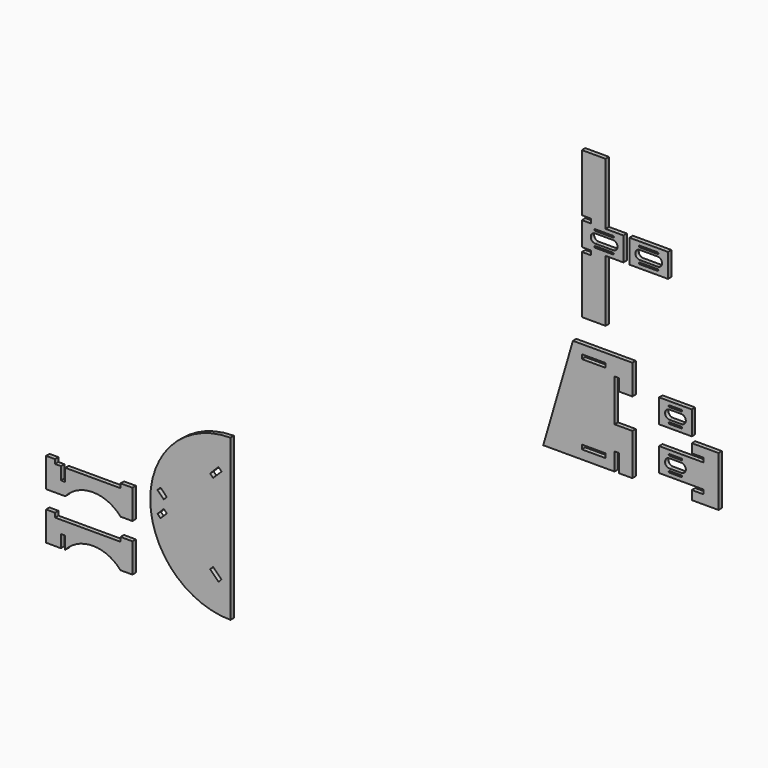
from build123d import *

# Parameters (mm, degrees)
F0_W     = 38.1
F0_H     = 18.288
F0_W_2   = 50.8
F0_W_3   = 18.288
F0_H_2   = 53.594
F1_DEPTH = 18.288
F0_W_4   = 101.6
F0_W_5   = 57.912
F0_H_3   = 76.2
F0_W_6   = 63.5
F0_W_7   = 139.7
F0_H_4   = 101.6
F0_W_8   = 165.1


# Not quite as in the source:
# - a feature names something its author has since deleted; it is built from what else it names


with BuildPart() as f1:
    # F0 (on Front) → F1 (new body)
    with BuildSketch(Plane.XZ):
        with Locations((-2420.2061958742, -155.956)):
            Rectangle(F0_W, F0_H)
        Polygon((-2401.1561958742, -165.1), (-2439.2561958742, -165.1), (-2439.2561958742, -272.288), (-2375.7561958742, -272.288), (-2375.7561958742, -218.694), (-2375.7561958742, -165.1), align=None)
        with BuildLine():
            Line((-2120.9, -165.1), (-2357.4681958742, -165.1))
            Line((-2357.4681958742, -165.1), (-2357.4681958742, -218.694))
            Line((-2357.4681958742, -218.694), (-2357.4681958742, -272.288))
            ThreePointArc((-2357.4681958742, -272.288), (-2239.1840979371, -218.694), (-2120.9, -272.288))
            Line((-2120.9, -272.288), (-2070.1, -272.288))
            Line((-2070.1, -272.288), (-2070.1, -165.1))
            Line((-2070.1, -165.1), (-2120.9, -165.1))
        make_face()
        with Locations((-2095.5, -155.956)):
            Rectangle(F0_W_2, F0_H)
        with Locations((-2366.6121958742, -245.491)):
            Rectangle(F0_W_3, F0_H_2)
    extrude(amount=F1_DEPTH)


with BuildPart() as f1b:
    # F0 (on Front) → F1, piece 2 (new body)
    with BuildSketch(Plane.XZ):
        with BuildLine():
            Line((-1651, -508), (-1651, 177.8))
            ThreePointArc((-1651, 177.8), (-1993.9, -165.1), (-1651, -508))
        make_face()
        Polygon((-1923.1920810565, -195.9920810565), (-1950.1328494197, -222.9328494197), (-1963.064418234, -210.0012806053), (-1936.1236498708, -183.0605122421), align=None, mode=Mode.SUBTRACT)
        Polygon((-1950.1328494197, -107.2671505803), (-1923.1920810565, -134.2079189435), (-1936.1236498708, -147.1394877579), (-1963.064418234, -120.1987193947), align=None, mode=Mode.SUBTRACT)
        Polygon((-1725.0210244843, -332.3789755157), (-1689.1, -368.3), (-1702.0315688143, -381.2315688143), (-1737.9525932986, -345.3105443301), align=None, mode=Mode.SUBTRACT)
        Polygon((-1702.0315688143, 51.0315688143), (-1689.1, 38.1), (-1725.0210244843, 2.1789755157), (-1737.9525932986, 15.1105443301), align=None, mode=Mode.SUBTRACT)
    extrude(amount=F1_DEPTH)


with BuildPart() as f1c:
    # F0 (on Front) → F1, piece 3 (new body)
    with BuildSketch(Plane.XZ):
        with Locations((-2420.2061958742, -357.632)):
            Rectangle(F0_W, F0_H)
        with BuildLine():
            Line((-2120.9, -366.776), (-2357.4681958742, -366.776))
            Line((-2357.4681958742, -366.776), (-2357.4681958742, -420.37))
            Line((-2357.4681958742, -420.37), (-2357.4681958742, -473.964))
            ThreePointArc((-2357.4681958742, -473.964), (-2239.1840979371, -420.37), (-2120.9, -473.964))
            Line((-2120.9, -473.964), (-2070.1, -473.964))
            Line((-2070.1, -473.964), (-2070.1, -366.776))
            Line((-2070.1, -366.776), (-2120.9, -366.776))
        make_face()
        with Locations((-2095.5, -357.632)):
            Rectangle(F0_W_2, F0_H)
        Polygon((-2401.1561958742, -366.776), (-2439.2561958742, -366.776), (-2439.2561958742, -473.964), (-2375.7561958742, -473.964), (-2375.7561958742, -420.37), (-2375.7561958742, -366.776), align=None)
        with Locations((-2366.6121958742, -393.573)):
            Rectangle(F0_W_3, F0_H_2)
    extrude(amount=F1_DEPTH)


with BuildPart() as f1d:
    # F0 (on Front) → F1, piece 4 (new body)
    with BuildSketch(Plane.XZ):
        Polygon((-98.044, 1503.6038), (-47.244, 1503.6038), (-47.244, 1748.8408), (-148.844, 1748.8408), (-148.844, 1503.6038), (-110.744, 1503.6038), align=None)
        Polygon((-98.044, 1485.3158), (-47.244, 1485.3158), (-47.244, 1503.6038), (-98.044, 1503.6038), (-110.744, 1503.6038), (-110.744, 1485.3158), align=None)
        Polygon((-98.044, 1383.7158), (-47.244, 1383.7158), (28.956, 1383.7158), (28.956, 1485.3158), (-47.244, 1485.3158), (-98.044, 1485.3158), (-110.744, 1485.3158), (-148.844, 1485.3158), (-148.844, 1383.7158), (-110.744, 1383.7158), align=None)
        with BuildLine():
            ThreePointArc((-91.694, 1399.4638), (-94.996, 1402.7658), (-91.694, 1406.0678))
            Line((-91.694, 1406.0678), (-15.494, 1406.0678))
            ThreePointArc((-15.494, 1406.0678), (-12.192, 1402.7658), (-15.494, 1399.4638))
            Line((-15.494, 1399.4638), (-91.694, 1399.4638))
        make_face(mode=Mode.SUBTRACT)
        with BuildLine():
            Line((-91.694, 1453.5658), (-15.494, 1453.5658))
            ThreePointArc((-15.494, 1453.5658), (3.556, 1434.5158), (-15.494, 1415.4658))
            Line((-15.494, 1415.4658), (-91.694, 1415.4658))
            ThreePointArc((-91.694, 1415.4658), (-110.744, 1434.5158), (-91.694, 1453.5658))
        make_face(mode=Mode.SUBTRACT)
        with BuildLine():
            Line((-15.494, 1462.9638), (-91.694, 1462.9638))
            ThreePointArc((-91.694, 1462.9638), (-94.996, 1466.2658), (-91.694, 1469.5678))
            Line((-91.694, 1469.5678), (-15.494, 1469.5678))
            ThreePointArc((-15.494, 1469.5678), (-12.192, 1466.2658), (-15.494, 1462.9638))
        make_face(mode=Mode.SUBTRACT)
        Polygon((-98.044, 1365.4278), (-47.244, 1365.4278), (-47.244, 1383.7158), (-98.044, 1383.7158), (-110.744, 1383.7158), (-110.744, 1365.4278), align=None)
        Polygon((-148.844, 1365.4278), (-148.844, 1120.1908), (-47.244, 1120.1908), (-47.244, 1365.4278), (-98.044, 1365.4278), (-110.744, 1365.4278), align=None)
    extrude(amount=F1_DEPTH)


with BuildPart() as f1e:
    # F0 (on Front) → F1, piece 5 (new body)
    with BuildSketch(Plane.XZ):
        Polygon((-9.144, 942.3908), (9.144, 942.3908), (9.144, 929.6908), (9.144, 891.5908), (67.056, 891.5908), (67.056, 929.6908), (67.056, 1018.5908), (-9.144, 1018.5908), (-186.944, 1018.5908), (-313.944, 584.2), (-9.144, 584.2), (-9.144, 660.4), (-9.144, 762), (-9.144, 929.6908), align=None)
        with Locations((-98.044, 631.444)):
            Rectangle(F0_W_4, F0_H, mode=Mode.SUBTRACT)
        with Locations((-98.044, 971.3468)):
            Rectangle(F0_W_4, F0_H, mode=Mode.SUBTRACT)
        Polygon((67.056, 762), (-9.144, 762), (-9.144, 660.4), (9.144, 660.4), (67.056, 660.4), align=None)
        with Locations((38.1, 622.3)):
            Rectangle(F0_W_5, F0_H_3)
    extrude(amount=F1_DEPTH)


with BuildPart() as f1f:
    # F0 (on Front) → F1, piece 6 (new body)
    with BuildSketch(Plane.XZ):
        Polygon((371.856, 760.476), (435.356, 760.476), (435.356, 798.576), (321.056, 798.576), (321.056, 760.476), align=None)
        with Locations((403.606, 751.332)):
            Rectangle(F0_W_6, F0_H)
        Polygon((181.356, 640.588), (371.856, 640.588), (435.356, 640.588), (435.356, 742.188), (371.856, 742.188), (181.356, 742.188), align=None)
        with BuildLine():
            ThreePointArc((276.606, 662.94), (279.908, 659.638), (276.606, 656.336))
            Line((276.606, 656.336), (225.806, 656.336))
            ThreePointArc((225.806, 656.336), (222.504, 659.638), (225.806, 662.94))
            Line((225.806, 662.94), (276.606, 662.94))
        make_face(mode=Mode.SUBTRACT)
        with BuildLine():
            Line((276.606, 672.338), (225.806, 672.338))
            ThreePointArc((225.806, 672.338), (206.756, 691.388), (225.806, 710.438))
            Line((225.806, 710.438), (276.606, 710.438))
            ThreePointArc((276.606, 710.438), (295.656, 691.388), (276.606, 672.338))
        make_face(mode=Mode.SUBTRACT)
        with BuildLine():
            Line((225.806, 726.44), (276.606, 726.44))
            ThreePointArc((276.606, 726.44), (279.908, 723.138), (276.606, 719.836))
            Line((276.606, 719.836), (225.806, 719.836))
            ThreePointArc((225.806, 719.836), (222.504, 723.138), (225.806, 726.44))
        make_face(mode=Mode.SUBTRACT)
        with Locations((403.606, 631.444)):
            Rectangle(F0_W_6, F0_H)
        Polygon((435.356, 622.3), (371.856, 622.3), (321.056, 622.3), (321.056, 584.2), (435.356, 584.2), align=None)
    extrude(amount=F1_DEPTH)


with BuildPart() as f1g:
    # F0 (on Front) → F1, piece 7 (new body)
    with BuildSketch(Plane.XZ):
        with Locations((251.206, 874.776)):
            Rectangle(F0_W_7, F0_H_4)
        with BuildLine():
            ThreePointArc((276.606, 846.328), (279.908, 843.026), (276.606, 839.724))
            Line((276.606, 839.724), (225.806, 839.724))
            ThreePointArc((225.806, 839.724), (222.504, 843.026), (225.806, 846.328))
            Line((225.806, 846.328), (276.606, 846.328))
        make_face(mode=Mode.SUBTRACT)
        with BuildLine():
            Line((276.606, 855.726), (225.806, 855.726))
            ThreePointArc((225.806, 855.726), (206.756, 874.776), (225.806, 893.826))
            Line((225.806, 893.826), (276.606, 893.826))
            ThreePointArc((276.606, 893.826), (295.656, 874.776), (276.606, 855.726))
        make_face(mode=Mode.SUBTRACT)
        with BuildLine():
            Line((276.606, 903.224), (225.806, 903.224))
            ThreePointArc((225.806, 903.224), (222.504, 906.526), (225.806, 909.828))
            Line((225.806, 909.828), (276.606, 909.828))
            ThreePointArc((276.606, 909.828), (279.908, 906.526), (276.606, 903.224))
        make_face(mode=Mode.SUBTRACT)
    extrude(amount=F1_DEPTH)


with BuildPart() as f1h:
    # F0 (on Front) → F1, piece 8 (new body)
    with BuildSketch(Plane.XZ):
        with Locations((136.906, 1434.5158)):
            Rectangle(F0_W_8, F0_H_4)
        with BuildLine():
            Line((98.806, 1406.0678), (175.006, 1406.0678))
            ThreePointArc((175.006, 1406.0678), (178.308, 1402.7658), (175.006, 1399.4638))
            Line((175.006, 1399.4638), (98.806, 1399.4638))
            ThreePointArc((98.806, 1399.4638), (95.504, 1402.7658), (98.806, 1406.0678))
        make_face(mode=Mode.SUBTRACT)
        with BuildLine():
            Line((175.006, 1415.4658), (98.806, 1415.4658))
            ThreePointArc((98.806, 1415.4658), (79.756, 1434.5158), (98.806, 1453.5658))
            Line((98.806, 1453.5658), (175.006, 1453.5658))
            ThreePointArc((175.006, 1453.5658), (194.056, 1434.5158), (175.006, 1415.4658))
        make_face(mode=Mode.SUBTRACT)
        with BuildLine():
            ThreePointArc((175.006, 1469.5678), (178.308, 1466.2658), (175.006, 1462.9638))
            Line((175.006, 1462.9638), (98.806, 1462.9638))
            ThreePointArc((98.806, 1462.9638), (95.504, 1466.2658), (98.806, 1469.5678))
            Line((98.806, 1469.5678), (175.006, 1469.5678))
        make_face(mode=Mode.SUBTRACT)
    extrude(amount=F1_DEPTH)


solid = Compound([f1.part, f1b.part, f1c.part, f1d.part, f1e.part, f1f.part, f1g.part, f1h.part])
